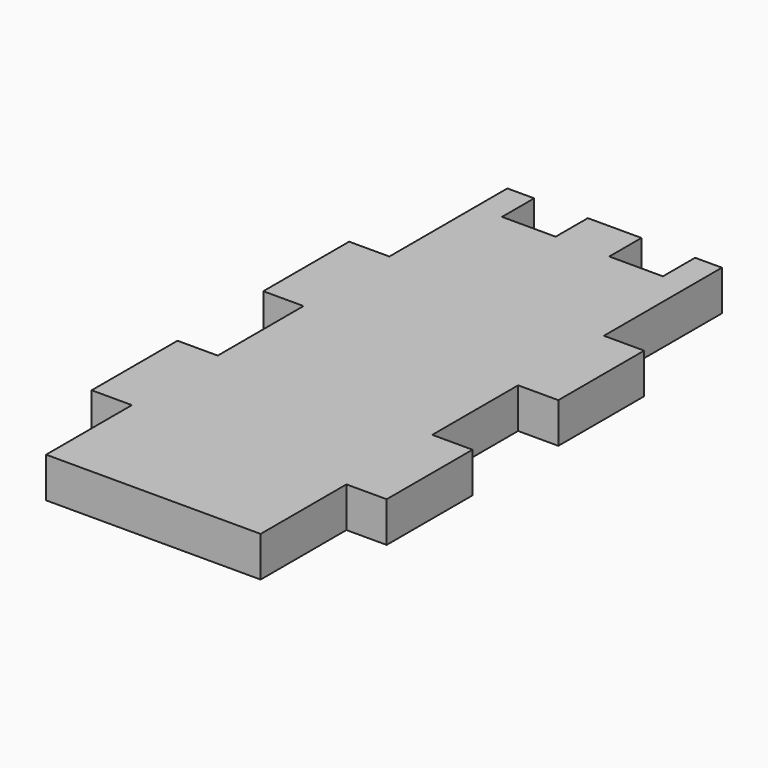
from build123d import *

# Parameters (mm, degrees)
F0_W     = 19.05
F0_H     = 50.8
F0_W_2   = 25.4
F0_H_2   = 19.05
F0_W_3   = 12.7
F1_DEPTH = 19.05


with BuildPart() as f1:
    # F0 (on Top) → F1 (new body)
    with BuildSketch(Plane.XY):
        with Locations((-111.125, 60.1353453214)):
            Rectangle(F0_W, F0_H)
        with Locations((-111.125, -41.4646546786)):
            Rectangle(F0_W, F0_H)
        Polygon((-88.9, 136.3353453214), (-101.6, 136.3353453214), (-101.6, 85.5353453214), (-101.6, 34.7353453214), (-101.6, -16.0646546786), (-101.6, -66.8646546786), (-101.6, -117.6646546786), (0, -117.6646546786), (0, -101.2241342793), (0, -66.8646546786), (0, -16.0646546786), (0, 34.7353453214), (0, 85.5353453214), (0, 136.3353453214), (-12.7, 136.3353453214), (-25.4, 136.3353453214), (-38.1, 136.3353453214), (-63.5, 136.3353453214), align=None)
        with Locations((9.525, -41.4646546786)):
            Rectangle(F0_W, F0_H)
        with Locations((9.525, 60.1353453214)):
            Rectangle(F0_W, F0_H)
        with Locations((-50.8, 145.8603453214)):
            Rectangle(F0_W_2, F0_H_2)
        with Locations((-95.25, 145.8603453214)):
            Rectangle(F0_W_3, F0_H_2)
        with Locations((-6.35, 145.8603453214)):
            Rectangle(F0_W_3, F0_H_2)
    extrude(amount=F1_DEPTH)


solid = f1.part
